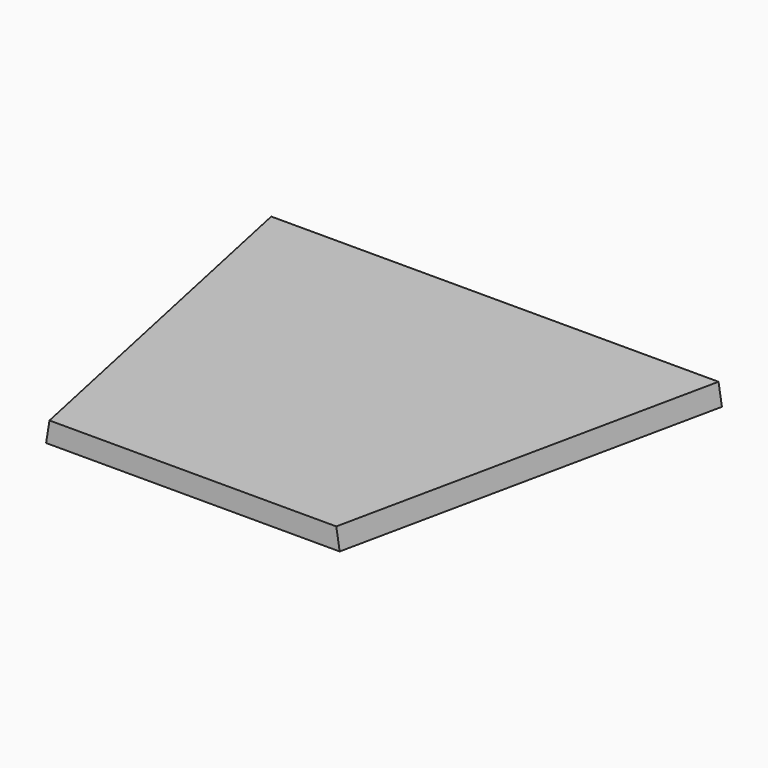
from build123d import *

# Parameters (mm, degrees)
F2_DEPTH   = 25.4
F3_SIZE2   = 4.022955
F3_SIZE    = 25.39999
F3_2_SIZE2 = 4.022955
F3_2_SIZE  = 25.39999


# Not quite as in the source:
# - a fillet or chamfer is up to 0.001 mm smaller than in the source, because OpenCascade refuses the exact size


with BuildPart() as f2:
    # F1 (on Top) → F2 (new body)
    with BuildSketch(Plane.XY):
        Polygon((-274.9808599955, 457.2), (-177.8, 0), (177.8, 0), (274.9808599955, 457.2), align=None)
    extrude(amount=F2_DEPTH)

    # F3 (size 25.4 and 4.0229647842 in the source; OpenCascade refuses exactly that, so slightly less here)
    f3_edges = [f2.edges().sort_by_distance(p)[0] for p in [
        (-226.39043, 228.6, 25.4),
    ]]
    f3_side = f2.faces().sort_by_distance((-226.39043, 228.6, 12.7))[0]
    chamfer(f3_edges, length=F3_SIZE, length2=F3_SIZE2, reference=f3_side)

    # F3#2 (size 25.4 and 4.0229647842 in the source; OpenCascade refuses exactly that, so slightly less here)
    f3_2_edges = [f2.edges().sort_by_distance(p)[0] for p in [
        (226.39043, 228.6, 25.4),
    ]]
    f3_2_side = f2.faces().sort_by_distance((226.39043, 228.6, 12.7))[0]
    chamfer(f3_2_edges, length=F3_2_SIZE, length2=F3_2_SIZE2, reference=f3_2_side)


solid = f2.part
